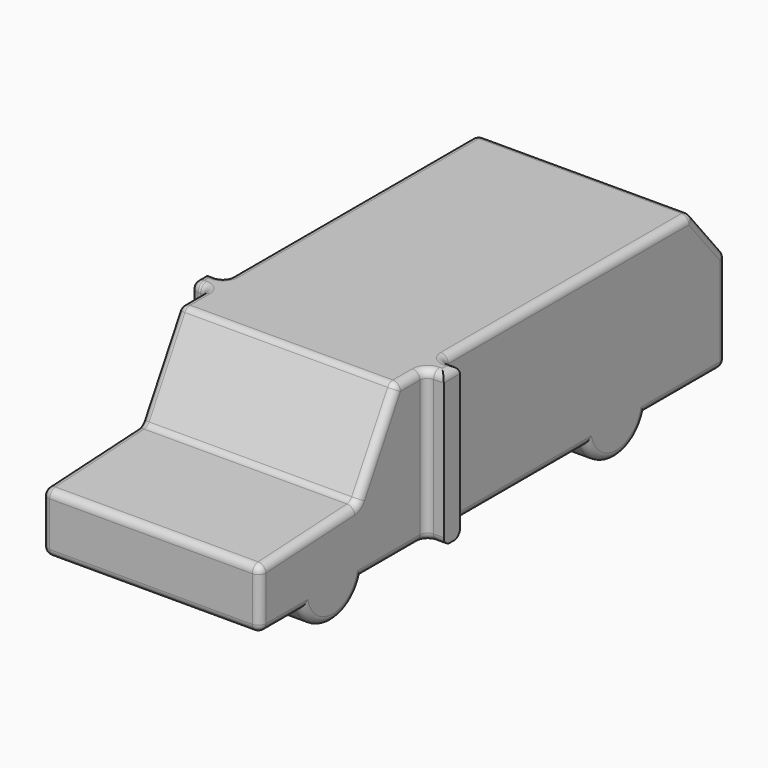
from build123d import *

# Parameters (mm, degrees)
F0_W     = 43
F0_H     = 70
F0_H_2   = 41
F0_H_3   = 4
F0_W_2   = 3.5
F1_DEPTH = 35
F2_W     = 133.2405284047
F2_H     = 49.6386280283
F2_W_2   = 4
F2_H_2   = 5.1434804872
F3_DEPTH = 71.3
F4_F1_R  = 1.5
F4_F2_R  = 1.5


with BuildPart() as f1:
    # F0 (on Top) → F1 (new body)
    with BuildSketch(Plane.XY):
        with Locations((0, 22.5)):
            Rectangle(F0_W, F0_H)
        with Locations((0, -37)):
            Rectangle(F0_W, F0_H_2)
        with Locations((0, -14.5)):
            Rectangle(F0_W, F0_H_3)
        with Locations((-23.25, -14.5)):
            Rectangle(F0_W_2, F0_H_3)
        with Locations((23.25, -14.5)):
            Rectangle(F0_W_2, F0_H_3)
    extrude(amount=F1_DEPTH)

    # F2 (on face) → F3 (cut)
    with BuildSketch(Plane(origin=(-25, 0, 0), x_dir=(0, -1, 0), z_dir=(-1, 0, 0))):
        with Locations((2.746347338, 15.9121430479)):
            Rectangle(F2_W, F2_H)
        with BuildLine():
            Line((-37.6789971831, 5.1434804872), (-57.6461282372, 5.1434804872))
            Line((-57.6461282372, 5.1434804872), (-57.6461282372, 24.5846966282))
            Line((-57.6461282372, 24.5846966282), (-48.9675998688, 35.1434804872))
            Line((-48.9675998688, 35.1434804872), (23.607192561, 35.1434804872))
            Line((23.607192561, 35.1434804872), (33.3717986941, 18.1189412251))
            Line((33.3717986941, 18.1189412251), (57.56669119, 16.8436886743))
            Line((57.56669119, 16.8436886743), (57.56669119, 5.1434804872))
            Line((57.56669119, 5.1434804872), (46.8123795631, 5.1434804872))
            ThreePointArc((46.8123795631, 5.1434804872), (39.56669119, 0.1434804872), (32.3210028169, 5.1434804872))
            Line((32.3210028169, 5.1434804872), (16.5, 5.1434804872))
            Line((16.5, 5.1434804872), (16.5, 0))
            Line((16.5, 0), (12.5, 0))
            Line((12.5, 0), (12.5, 5.1434804872))
            Line((12.5, 5.1434804872), (-23.1876204369, 5.1434804872))
            ThreePointArc((-23.1876204369, 5.1434804872), (-30.43330881, 0.1434804872), (-37.6789971831, 5.1434804872))
        make_face(mode=Mode.SUBTRACT)
        with Locations((14.5, 2.5717402436)):
            Rectangle(F2_W_2, F2_H_2)
    extrude(amount=-F3_DEPTH, mode=Mode.SUBTRACT)

    # F4: fillet of radius 1.5 on 46 edges, made by hand

    # F4_f1
    f4_f1_edges = [f1.edges().sort_by_distance(p)[0] for p in [
        (0, -33.3717986941, 18.1189412251),
        (21.5, -16.5, 20.0717402436),
        (-21.5, -16.5, 20.0717402436),
        (-21.5, -12.5, 20.0717402436),
        (21.5, -12.5, 20.0717402436),
    ]]
    fillet(f4_f1_edges, radius=F4_F1_R)

    # F4_f2
    f4_f2_edges = [f1.edges().sort_by_distance(p)[0] for p in [
        (-21.5, 19.0427650337, 35),
        (-21.5, -28.3274234666, 26.9137828136),
        (0, -23.6894873253, 35),
        (-21.5, -20.8447436626, 35),
        (0, -57.5, 16.8472038009),
        (21.5, -52.1561897815, 5.1434804872),
        (21.5, -39.56669119, 0.1434804872),
        (21.5, -25.1605014085, 5.1434804872),
        (21.5, -20.8447436626, 35),
        (21.5, -28.3274234666, 26.9137828136),
        (21.5, -45.8437879598, 17.4615737196),
        (21.5, -57.5, 10.995342144),
        (0, -57.5, 5.1434804872),
        (-24, -16.5, 35),
        (-25, -16.5, 20.0717402436),
        (-24, -16.5, 5.1434804872),
        (-25, -14.5, 5.1434804872),
        (-21.5, 47.5894985915, 5.1434804872),
        (-21.5, 30.43330881, 0.1434804872),
        (-21.5, 6.0938102185, 5.1434804872),
        (-21.5, 53.2927650337, 29.8812422145),
        (-21.5, 57.5, 14.9529824581),
        (21.5, 19.0427650337, 35),
        (24, -12.5, 35),
        (25, -14.5, 35),
        (24, -16.5, 35),
        (-25, -14.5, 35),
        (-24, -12.5, 35),
        (0, 49.0855300674, 35),
        (21.5, 6.0938102185, 5.1434804872),
        (21.5, 30.43330881, 0.1434804872),
        (21.5, 47.5894985915, 5.1434804872),
        (21.5, 57.5, 14.9529824581),
        (21.5, 53.2927650337, 29.8812422145),
        (0, 57.5, 24.762484429),
        (0, 57.5, 5.1434804872),
        (-21.5, -25.1605014085, 5.1434804872),
        (-21.5, -39.56669119, 0.1434804872),
        (-21.5, -52.1561897815, 5.1434804872),
        (-21.5, -57.5, 10.995342144),
        (-21.5, -45.8437879598, 17.4615737196),
        (-21.5, -33.4807690606, 18.2961384884),
        (-21.9393398282, -16.9393398282, 5.1434804872),
        (21.9393398282, -12.0606601718, 5.1434804872),
        (-21.9393398282, -12.0606601718, 35),
        (21.9393398282, -16.9393398282, 35),
        (21.9393398282, -12.0606601718, 35),
        (-21.9393398282, -12.0606601718, 5.1434804872),
        (-21.9393398282, -16.9393398282, 35),
        (21.5, -33.4807690606, 18.2961384884),
        (21.9393398282, -16.9393398282, 5.1434804872),
    ]]
    fillet(f4_f2_edges, radius=F4_F2_R)


solid = f1.part
